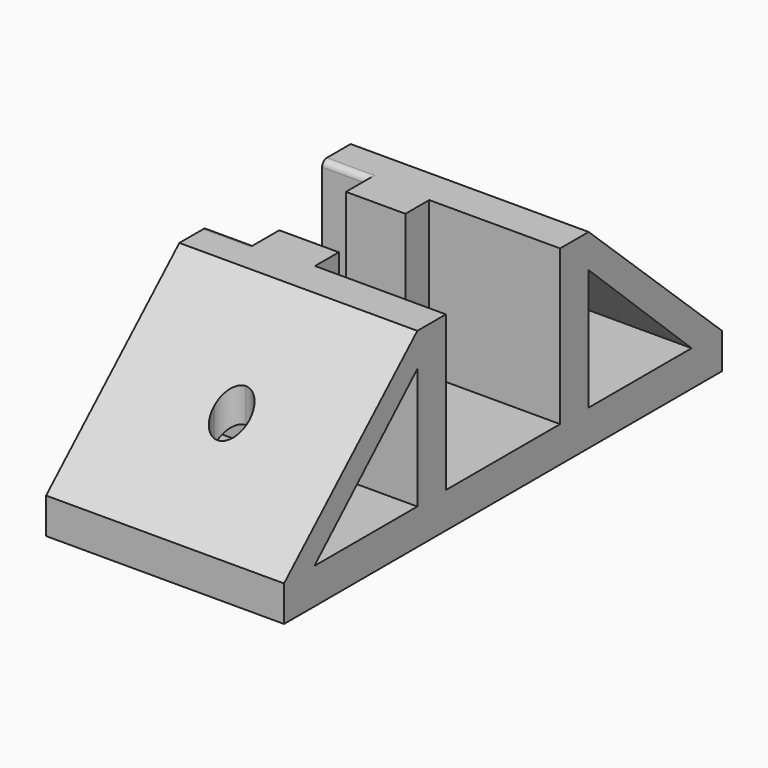
from build123d import *

# Parameters (mm, degrees)
F0_W      = 20
F0_H      = 46
F1_DEPTH  = 3
F2_W      = 20
F2_H      = 3
F3_DEPTH  = 13
F6_DEPTH  = 25
F7_DEPTH  = 25
F9_DEPTH  = 20
F11_DEPTH = 20
F12_DEPTH = 25
F13_DEPTH = 25
F14_W     = 5
F14_H     = 12
F15_DEPTH = 13
F17_DEPTH = 25
F18_R     = 0.5


# Not quite as in the source:
# - ends of sketch curves that miss each other by under 0.0002 mm in the source are joined


with BuildPart() as f1:
    # F0 (on Top) → F1 (new body)
    with BuildSketch(Plane.XY):
        with Locations((10, -23)):
            Rectangle(F0_W, F0_H)
    extrude(amount=F1_DEPTH)

    # F2 (on face) → F3 (join)
    with BuildSketch(Plane.XY.offset(3)):
        with Locations((10, -15.5)):
            Rectangle(F2_W, F2_H)
        with Locations((10, -30.5)):
            Rectangle(F2_W, F2_H)
    extrude(amount=F3_DEPTH)

    # F5 (on face) → F6 (cut)
    with BuildSketch(Plane.XY.offset(3)):
        with BuildLine():
            Line((10, -39), (8.5, -39))
            ThreePointArc((8.5, -39), (10, -40.5), (11.5, -39))
            ThreePointArc((11.5, -39), (11.0606601718, -37.9393398282), (10, -37.5))
            Line((10, -37.5), (10, -39))
        make_face()
        with BuildLine():
            ThreePointArc((10, -37.5), (8.9393398282, -37.9393398282), (8.5, -39))
            Line((8.5, -39), (10, -39))
            Line((10, -39), (10, -37.5))
        make_face()
    extrude(amount=-F6_DEPTH, mode=Mode.SUBTRACT)

    # F5 (on face) → F7 (cut)
    with BuildSketch(Plane.XY.offset(3)):
        with BuildLine():
            ThreePointArc((11.5000007078, -7), (11.0606608796, -5.9393398282), (10.0000007078, -5.5))
            Line((10.0000007078, -5.5), (10.0000007078, -7))
            Line((10.0000007078, -7), (10, -8.5))
            ThreePointArc((10, -8.5), (11.0606606293, -8.060660422), (11.5000007078, -7))
        make_face()
        with BuildLine():
            Line((10.0000007078, -7), (8.5000007078, -7))
            ThreePointArc((8.5000007078, -7), (8.9393402858, -8.0606599215), (10, -8.5))
            Line((10, -8.5), (10.0000007078, -7))
        make_face()
        with BuildLine():
            Line((10.0000007078, -7), (10.0000007078, -5.5))
            ThreePointArc((10.0000007078, -5.5), (8.939340536, -5.9393398282), (8.5000007078, -7))
            Line((8.5000007078, -7), (10.0000007078, -7))
        make_face()
    extrude(amount=-F7_DEPTH, mode=Mode.SUBTRACT)

    # F8 (on face) → F9 (join)
    with BuildSketch(Plane(origin=(0, 0, 0), x_dir=(0, -1, 0), z_dir=(-1, 0, 0))):
        Polygon((46, 3), (32, 16), (29, 16), (46, 0), align=None)
    extrude(amount=-F9_DEPTH)

    # F10 (on face) → F11 (join)
    with BuildSketch(Plane.YZ.offset(20)):
        Polygon((0, 3), (-14, 16), (-14, 13.1764705882), (-3.1875, 3), align=None)
    extrude(amount=-F11_DEPTH)

    # F5 (on face) → F12 (cut)
    with BuildSketch(Plane.XY.offset(3)):
        with BuildLine():
            Line((10, -39), (8.5, -39))
            ThreePointArc((8.5, -39), (10, -40.5), (11.5, -39))
            ThreePointArc((11.5, -39), (11.0606601718, -37.9393398282), (10, -37.5))
            Line((10, -37.5), (10, -39))
        make_face()
        with BuildLine():
            ThreePointArc((10, -37.5), (8.9393398282, -37.9393398282), (8.5, -39))
            Line((8.5, -39), (10, -39))
            Line((10, -39), (10, -37.5))
        make_face()
    extrude(amount=F12_DEPTH, mode=Mode.SUBTRACT)

    # F5 (on face) → F13 (cut)
    with BuildSketch(Plane.XY.offset(3)):
        with BuildLine():
            ThreePointArc((11.5000007078, -7), (11.0606608796, -5.9393398282), (10.0000007078, -5.5))
            Line((10.0000007078, -5.5), (10.0000007078, -7))
            Line((10.0000007078, -7), (10, -8.5))
            ThreePointArc((10, -8.5), (11.0606606293, -8.060660422), (11.5000007078, -7))
        make_face()
        with BuildLine():
            Line((10.0000007078, -7), (8.5000007078, -7))
            ThreePointArc((8.5000007078, -7), (8.9393402858, -8.0606599215), (10, -8.5))
            Line((10, -8.5), (10.0000007078, -7))
        make_face()
        with BuildLine():
            Line((10.0000007078, -7), (10.0000007078, -5.5))
            ThreePointArc((10.0000007078, -5.5), (8.939340536, -5.9393398282), (8.5000007078, -7))
            Line((8.5000007078, -7), (10.0000007078, -7))
        make_face()
    extrude(amount=F13_DEPTH, mode=Mode.SUBTRACT)

    # F14 (on face) → F15 (join)
    with BuildSketch(Plane.XY.offset(3)):
        with Locations((6.5, -23)):
            Rectangle(F14_W, F14_H)
    extrude(amount=F15_DEPTH)

    # F16 (on face) → F17 (cut)
    with BuildSketch(Plane(origin=(4, 0, 0), x_dir=(0, -1, 0), z_dir=(-1, 0, 0))):
        with BuildLine():
            Line((19.5, 16), (19.5, 9))
            ThreePointArc((19.5, 9), (23, 12.5), (26.5, 9))
            Line((26.5, 9), (26.5, 16))
            Line((26.5, 16), (19.5, 16))
        make_face()
        with BuildLine():
            ThreePointArc((26.5, 9), (23, 12.5), (19.5, 9))
            Line((19.5, 9), (23, 9))
            Line((23, 9), (26.5, 9))
        make_face()
        with BuildLine():
            ThreePointArc((19.5, 9), (20.5251262658, 6.5251262658), (23, 5.5))
            Line((23, 5.5), (23, 9))
            Line((23, 9), (19.5, 9))
        make_face()
        with BuildLine():
            Line((23, 9), (23, 5.5))
            ThreePointArc((23, 5.5), (25.4748737342, 6.5251262658), (26.5, 9))
            Line((26.5, 9), (23, 9))
        make_face()
    extrude(amount=-F17_DEPTH, mode=Mode.SUBTRACT)

    # F18
    f18_edges = [f1.edges().sort_by_distance(p)[0] for p in [
        (2, -17, 16),
        (2, -29, 16),
    ]]
    fillet(f18_edges, radius=F18_R)


solid = f1.part
